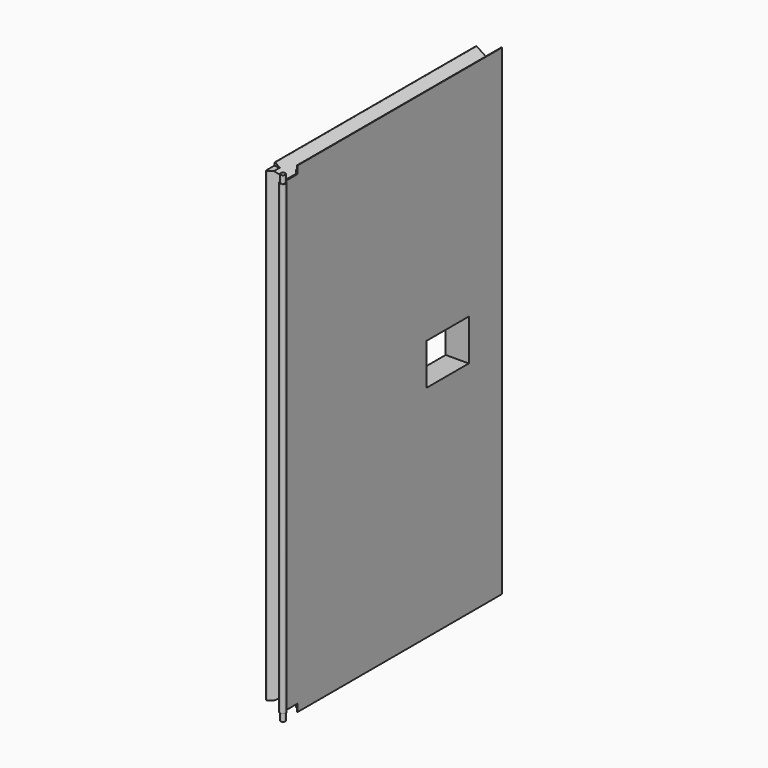
from build123d import *

# Parameters (mm, degrees)
F1_DEPTH       = 0.889
F3_DEPTH       = 38.1
F5_DEPTH       = 450.851
F7_DEPTH       = 806.451
F8_R           = 1.27
F9_R           = 1.27
F10_W          = 88.9
F10_H          = 34.925
F11_DEPTH      = 38.99
F12_R          = 5.03555
F12_R_2        = 3.96875
F13_DEPTH      = 393.7
F13_DEPTH_BACK = 393.7
F14_R          = 3.96875
F15_DEPTH      = 406.4
F15_DEPTH_BACK = 406.4


with BuildPart() as f1:
    # F0 (on Right) → F1 (new body)
    with BuildSketch(Plane.YZ):
        Polygon((228.6, 406.4), (-203.2, 406.4), (-203.2, 393.7), (-228.6, 393.7), (-228.6, 0), (228.6, 0), align=None)
        Polygon((228.6, -406.4), (228.6, 0), (-228.6, 0), (-228.6, -393.7), (-203.2, -393.7), (-203.2, -406.4), align=None)
    extrude(amount=-F1_DEPTH)

    # F2 (on face) → F3 (join)
    with BuildSketch(Plane(origin=(-0.889, 0, 0), x_dir=(0, -1, 0), z_dir=(-1, 0, 0))):
        Polygon((203.2, 400.05), (-222.25, 400.05), (-222.25, -400.05), (203.2, -400.05), (203.2, -393.7), (222.25, -393.7), (222.25, 393.7), (203.2, 393.7), align=None)
    extrude(amount=F3_DEPTH)

    # F4 (on face) → F5 (cut, through all)
    with BuildSketch(Plane(origin=(0, 222.25, 0), x_dir=(-1, 0, 0), z_dir=(0, 1, 0))):
        Polygon((2.1336, -400.05), (38.989, -400.05), (2.1336, -375.200815087), align=None)
        Polygon((2.1336, 375.200815087), (38.989, 400.05), (2.1336, 400.05), align=None)
    extrude(amount=-F5_DEPTH, mode=Mode.SUBTRACT)

    # F6 (on face) → F7 (cut, through all)
    with BuildSketch(Plane.XY.offset(400.05)):
        Polygon((-2.1336, 247.099184913), (-38.989, 222.25), (-2.1336, 222.25), align=None)
        Polygon((-2.1336, -203.2), (-2.1336, -197.400815087), (-38.989, -222.25), (-2.1336, -222.25), align=None)
    extrude(amount=-F7_DEPTH, mode=Mode.SUBTRACT)

    # F8
    f8_edges = [f1.edges().sort_by_distance(p)[0] for p in [
        (-38.989, 9.525, -400.05),
        (-38.989, 222.25, 0),
        (-38.989, 9.525, 400.05),
        (-38.989, -222.25, 0),
    ]]
    fillet(f8_edges, radius=F8_R)

    # F9
    f9_edges = [f1.edges().sort_by_distance(p)[0] for p in [
        (-2.1336, 12.424592, 375.200815),
        (-2.1336, 12.424592, -375.200815),
    ]]
    fillet(f9_edges, radius=F9_R)

    # F10 (on face) → F11 (cut, through all)
    with BuildSketch(Plane.YZ):
        with Locations((114.3, 17.4625)):
            Rectangle(F10_W, F10_H)
        with Locations((114.3, -17.4625)):
            Rectangle(F10_W, F10_H)
    extrude(amount=-F11_DEPTH, mode=Mode.SUBTRACT)


with BuildPart() as f13:
    # F12 (on Top) → F13 (new body, two sides)
    with BuildSketch(Plane.XY) as f13_sk:
        with Locations((0, -233.63555)):
            Circle(F12_R)
        with Locations((0, -233.63555)):
            Circle(F12_R_2, mode=Mode.SUBTRACT)
    extrude(amount=F13_DEPTH)
    extrude(f13_sk.sketch, amount=-F13_DEPTH_BACK)

    # F14 (on Top) → F15 (join, two sides)
    with BuildSketch(Plane.XY) as f15_sk:
        with Locations((0, -233.63555)):
            Circle(F14_R)
    extrude(amount=F15_DEPTH)
    extrude(f15_sk.sketch, amount=-F15_DEPTH_BACK)


solid = Compound([f1.part, f13.part])
